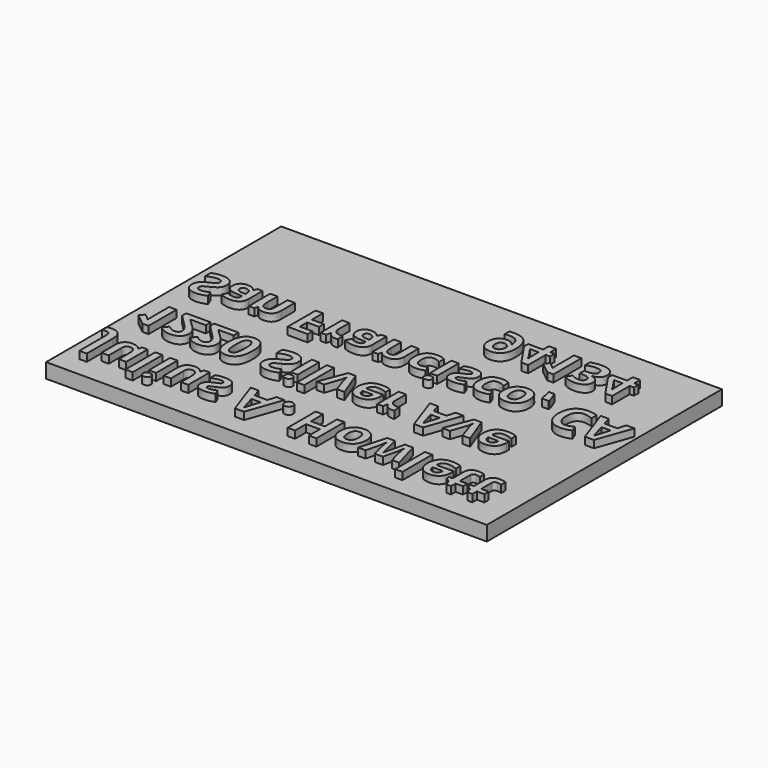
from build123d import *

# Parameters (mm, degrees)
F0_W         = 60
F0_H         = 40
F1_DEPTH     = 2
F3_TEXT_SIZE = 6.675822743
F4_DEPTH     = 1


# Not quite as in the source:
# - Text() gives the source's letters only with a copy of the font that has no kerning and outlines rounded to 1/6400 em; it was checked with that copy


with BuildPart() as f1:
    # F0 (on Top) → F1 (new body)
    with BuildSketch(Plane.XY):
        Rectangle(F0_W, F0_H)
    extrude(amount=F1_DEPTH)

    # F3 (on offset) → F4 (join)
    with BuildSketch(Plane(origin=(0, 0, 2), x_dir=(1, 0, 0), z_dir=(0, 0, -1))):
        with Locations((-28.2653291841, 12.4915869696)):
            Text('Julius A. Howlett', F3_TEXT_SIZE, font='Open Sans', font_style=FontStyle.BOLD, text_align=(TextAlign.LEFT, TextAlign.BOTTOM))
        with Locations((-28.2653291841, 3.4124680391)):
            Text('1220 Silver Ave', F3_TEXT_SIZE, font='Open Sans', font_style=FontStyle.BOLD, text_align=(TextAlign.LEFT, TextAlign.BOTTOM))
        with Locations((-28.2653291841, -5.6666508914)):
            Text('San Francisco, CA', F3_TEXT_SIZE, font='Open Sans', font_style=FontStyle.BOLD, text_align=(TextAlign.LEFT, TextAlign.BOTTOM))
        with Locations((4.6934163175, -14.7457698219)):
            Text('94134', F3_TEXT_SIZE, font='Open Sans', font_style=FontStyle.BOLD, text_align=(TextAlign.LEFT, TextAlign.BOTTOM))
    extrude(amount=-F4_DEPTH)


solid = f1.part
